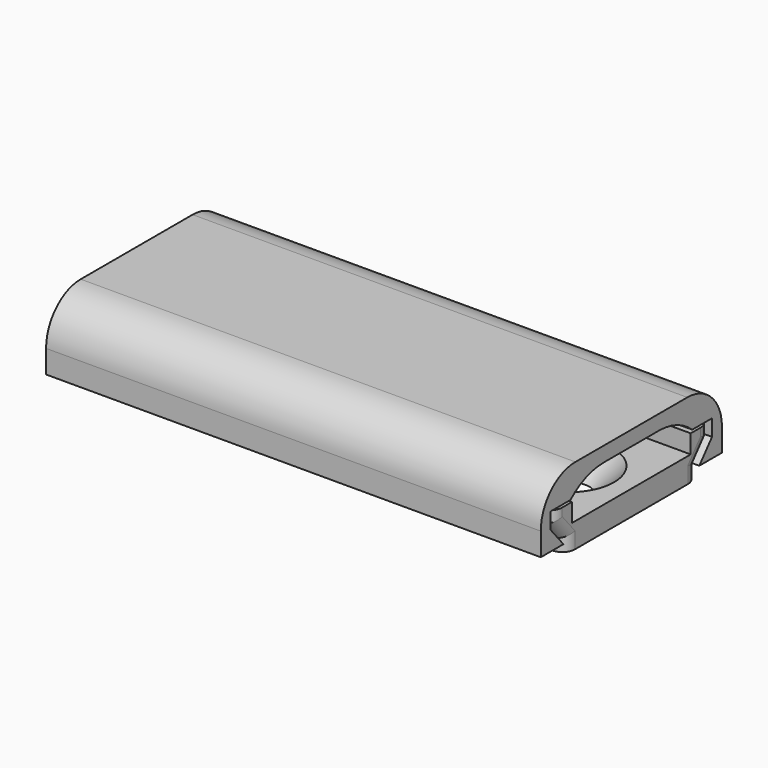
from build123d import *

# Parameters (mm, degrees)
F1_W         = 40
F1_H         = 12
F1_R         = 1.6
F2_DEPTH     = 2
F1_H_2       = 2
F3_DEPTH     = 3.5
F5_DEPTH     = 282.2
F7_DEPTH     = 40
F8_R         = 1
F9_SIZE      = 1.99999
F10_T1_DEPTH = 40
F11_R        = 3.5


# Not quite as in the source:
# - a fillet or chamfer that OpenCascade refuses, or shapes differently, is made with other operations: its cross-section is extruded or revolved along the edge and cut away or added
# - a fillet or chamfer is up to 0.001 mm smaller than in the source, because OpenCascade refuses the exact size


with BuildPart() as f2:
    # F1 (on Top) → F2 (new body)
    with BuildSketch(Plane.XY):
        Rectangle(F1_W, F1_H)
        with Locations((-15, 0)):
            Circle(F1_R, mode=Mode.SUBTRACT)
        Circle(F1_R, mode=Mode.SUBTRACT)
        with Locations((15, 0)):
            Circle(F1_R, mode=Mode.SUBTRACT)
    extrude(amount=F2_DEPTH)

    # F1 (on Top) → F3 (join)
    with BuildSketch(Plane.XY):
        with Locations((0, 7)):
            Rectangle(F1_W, F1_H_2)
        with Locations((0, -7)):
            Rectangle(F1_W, F1_H_2)
    extrude(amount=F3_DEPTH)

    # F4 (on face) → F5 (cut)
    with BuildSketch(Plane(origin=(-20, 0, 0), x_dir=(0, -1, 0), z_dir=(-1, 0, 0))):
        Polygon((-6.7144247806, 0.9679111138), (-8, 2.5), (-8, 0), (-6.7144247806, 0), align=None)
        Polygon((6.7144247806, 0.9679111138), (6.7144247806, 0), (8, 0), (8, 2.5), align=None)
    extrude(amount=-F5_DEPTH, mode=Mode.SUBTRACT)

    # F8
    f8_edges = [f2.edges().sort_by_distance(p)[0] for p in [
        (20, -8, 3),
        (20, -6.714425, 0.483956),
        (20, -7.357212, 1.733956),
        (20, 8, 3),
        (20, 7.357212, 1.733956),
        (20, 6.714425, 0.483956),
        (-20, 8, 3),
        (-20, 7.357212, 1.733956),
        (-20, 6.714425, 0.483956),
        (-20, -7.357212, 1.733956),
        (-20, -6.714425, 0.483956),
        (-20, -8, 3),
    ]]
    fillet(f8_edges, radius=F8_R)

    # F9 (size 2 in the source; OpenCascade refuses exactly that, so slightly less here)
    f9_edges = [f2.edges().sort_by_distance(p)[0] for p in [
        (-16.6, 0, 2),
        (-1.6, 0, 2),
        (13.4, 0, 2),
    ]]
    chamfer(f9_edges, length=F9_SIZE)


with BuildPart() as f7:
    # F6 (on face) → F7 (new body)
    with BuildSketch(Plane(origin=(-20, 0, 0), x_dir=(0, -1, 0), z_dir=(-1, 0, 0))):
        Polygon((-6.8676336693, 0.8393535918), (-8.1532088886, 2.3714424781), (-8.1532088886, 3.7), (-8.1532088886, 5), (-7.2440384092, 5), (0, 5), (7.2440384092, 5), (8.1532088886, 5), (8.1532088886, 3.7), (8.1532088886, 2.3714424781), (6.8676336693, 0.8393535918), (9.1532088886, 0.8393535918), (9.1532088886, 6.2), (0, 6.2), (-9.1532088886, 6.2), (-9.1532088886, 0.8393535918), align=None)
        Polygon((-8.1532088886, 5), (-8.1532088886, 3.7), (-6.1532088886, 3.7), (-7.2440384092, 5), align=None)
        Polygon((8.1532088886, 5), (7.2440384092, 5), (6.1532088886, 3.7), (8.1532088886, 3.7), align=None)
    extrude(amount=-F7_DEPTH)

    # F10: fillet of radius 5 on 2 edges, made by hand

    # F10_s2 → F10_t1 (join)
    with BuildSketch(Plane.YZ.offset(-20)):
        with BuildLine():
            ThreePointArc((6.1532088886, 3.7), (4.5929501822, 4.6636895265), (2.7901745445, 5))
            Line((2.7901745445, 5), (7.2440384092, 5))
            Line((7.2440384092, 5), (6.1532088886, 3.7))
        make_face()
        with BuildLine():
            ThreePointArc((-2.7901745445, 5), (-4.5929501822, 4.6636895265), (-6.1532088886, 3.7))
            Line((-6.1532088886, 3.7), (-7.2440384092, 5))
            Line((-7.2440384092, 5), (-2.7901745445, 5))
        make_face()
    extrude(amount=F10_T1_DEPTH)

    # F11
    f11_edges = [f7.edges().sort_by_distance(p)[0] for p in [
        (0, -9.153209, 6.2),
        (0, 9.153209, 6.2),
    ]]
    fillet(f11_edges, radius=F11_R)


solid = Compound([f2.part, f7.part])
